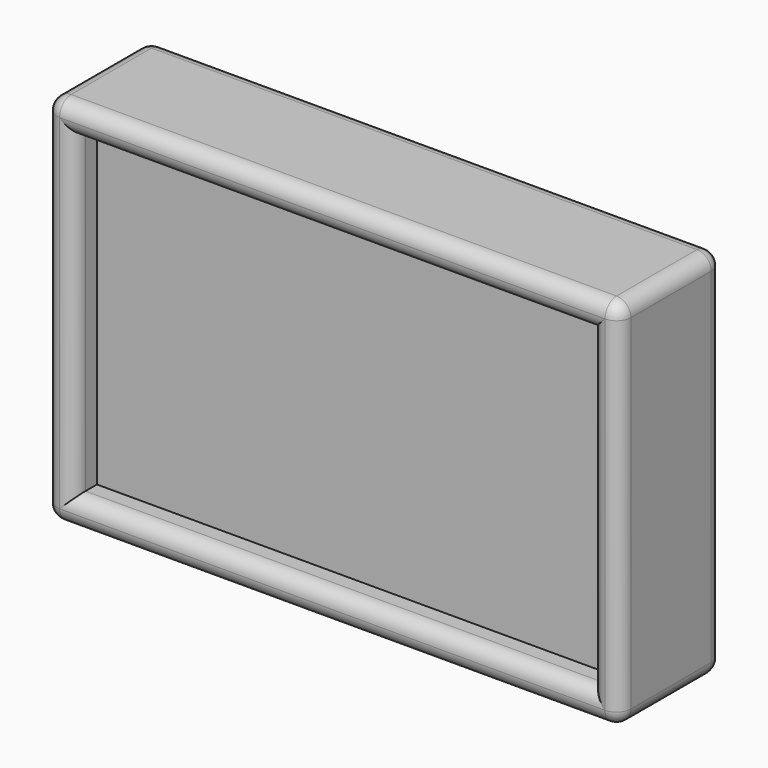
from build123d import *

# Parameters (mm, degrees)
F0_W     = 180
F0_H     = 110
F1_DEPTH = 35
F0_W_2   = 200
F0_H_2   = 130
F2_DEPTH = 45
F3_R     = 4.99999


# Not quite as in the source:
# - a fillet or chamfer is up to 0.001 mm smaller than in the source, because OpenCascade refuses the exact size


with BuildPart() as f1:
    # F0 (on Front) → F1 (new body)
    with BuildSketch(Plane.XZ):
        Rectangle(F0_W, F0_H)
    extrude(amount=F1_DEPTH)

    # F0 (on Front) → F2 (join)
    with BuildSketch(Plane.XZ):
        Rectangle(F0_W_2, F0_H_2)
        Rectangle(F0_W, F0_H, mode=Mode.SUBTRACT)
    extrude(amount=F2_DEPTH)

    # F3 (radius 5 in the source; OpenCascade refuses exactly that, so slightly less here)
    f3_edges = [f1.edges().sort_by_distance(p)[0] for p in [
        (0, -45, -65),
        (100, -45, 0),
        (0, -45, 65),
        (-100, -45, 0),
        (0, -45, 55),
        (90, -45, 0),
        (0, -45, -55),
        (-90, -45, 0),
        (-100, -22.5, -65),
        (100, -22.5, -65),
        (0, 0, -65),
        (-100, -22.5, 65),
        (-100, 0, 0),
        (100, -22.5, 65),
        (100, 0, 0),
        (0, 0, 65),
    ]]
    fillet(f3_edges, radius=F3_R)


solid = f1.part
